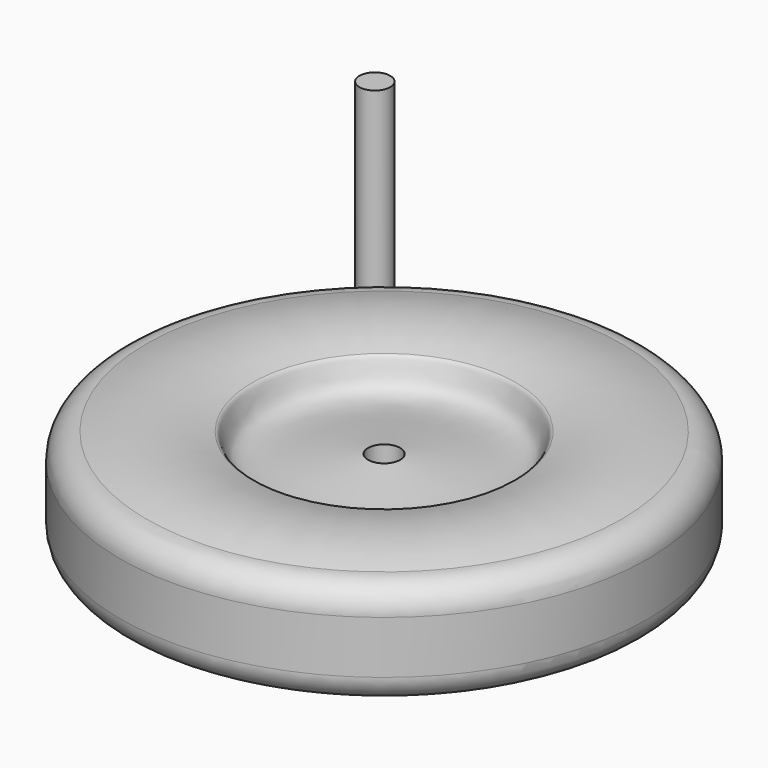
from build123d import *

# Parameters (mm, degrees)
F0_R     = 1.75
F1_DEPTH = 30
F6_D     = 3.6576


# Not quite as in the source:
# - a fillet or chamfer that OpenCascade refuses, or shapes differently, is made with other operations: its cross-section is extruded or revolved along the edge and cut away or added


with BuildPart() as f1:
    # F0 (on Top) → F1 (new body)
    with BuildSketch(Plane.XY):
        with Locations((-21.0584960878, 25.0069648027)):
            Circle(F0_R)
    extrude(amount=F1_DEPTH)


with BuildPart() as f3:
    # F2 (on Front) → F3 (revolve)
    with BuildSketch(Plane.XZ):
        with BuildLine():
            Line((0, 10), (0, 0))
            Line((0, 0), (6, 0))
            Line((6, 0), (6, 2))
            Line((6, 2), (15, 2))
            Line((15, 2), (15, 0))
            Line((15, 0), (27, 0))
            ThreePointArc((27, 0), (29.1213203436, 0.8786796564), (30, 3))
            Line((30, 3), (30, 9))
            ThreePointArc((30, 9), (29.1213203436, 11.1213203436), (27, 12))
            ThreePointArc((27, 12), (21, 12.9280272043), (15, 12))
            add(Edge.make_bspline(
                [(0, 10), (3.294109879, 9.5346706659), (7.2319046155, 9.1457099045), (14.3270360542, 8.1327705449), (14.4332102752, 11.8877358395), (15, 12)],
                knots=[0, 0, 0, 0, 0.4115020239, 0.7567346673, 1, 1, 1, 1], degree=3))
        make_face()
    revolve(axis=Axis((0, 0, 5), (0, 0, 1)))

    # F4: fillet of radius 5 on 1 edges, made by hand

    # F4_s1 → F4_t2 (revolve, cut)
    with BuildSketch(Plane.XZ):
        with BuildLine():
            ThreePointArc((15, 2), (16.7639320225, 0.527864045), (19, 0))
            Line((19, 0), (15, 0))
            Line((15, 0), (15, 2))
        make_face()
    revolve(axis=Axis((0, 0, 0), (0, 0, 1)), mode=Mode.SUBTRACT)

    # F6 (through all)
    with Locations(Plane(origin=(0, 0, 0), x_dir=(1, 0, 0), z_dir=(0, 0, -1))):
        with Locations((0, 0)):
            Hole(F6_D / 2)


solid = Compound([f1.part, f3.part])
